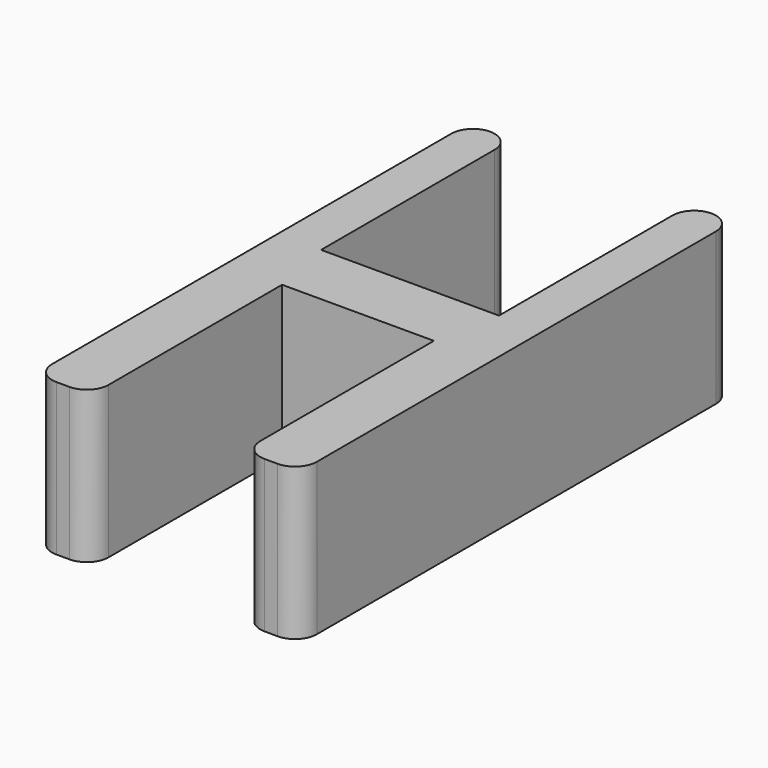
from build123d import *

# Parameters (mm, degrees)
F1_DEPTH = 7
F2_R     = 0.99999


# Not quite as in the source:
# - a fillet or chamfer is up to 0.001 mm smaller than in the source, because OpenCascade refuses the exact size


with BuildPart() as f1:
    # F0 (on Top) → F1 (new body)
    with BuildSketch(Plane.XY):
        Polygon((4.1, 1.5), (0, 1.5), (-4.1, 1.5), (-4.1, 12.5), (-6.1, 12.5), (-6.1, -12.5), (-3.5, -12.5), (-3.5, -1.5), (0, -1.5), (3.5, -1.5), (3.5, -12.5), (6.1, -12.5), (6.1, 12.5), (4.1, 12.5), align=None)
    extrude(amount=F1_DEPTH)

    # F2 (radius 1 in the source; OpenCascade refuses exactly that, so slightly less here)
    f2_edges = [f1.edges().sort_by_distance(p)[0] for p in [
        (3.5, -12.5, 3.5),
        (6.1, -12.5, 3.5),
        (-3.5, -12.5, 3.5),
        (-6.1, -12.5, 3.5),
        (6.1, 12.5, 3.5),
        (4.1, 12.5, 3.5),
        (-4.1, 12.5, 3.5),
        (-6.1, 12.5, 3.5),
    ]]
    fillet(f2_edges, radius=F2_R)


solid = f1.part
